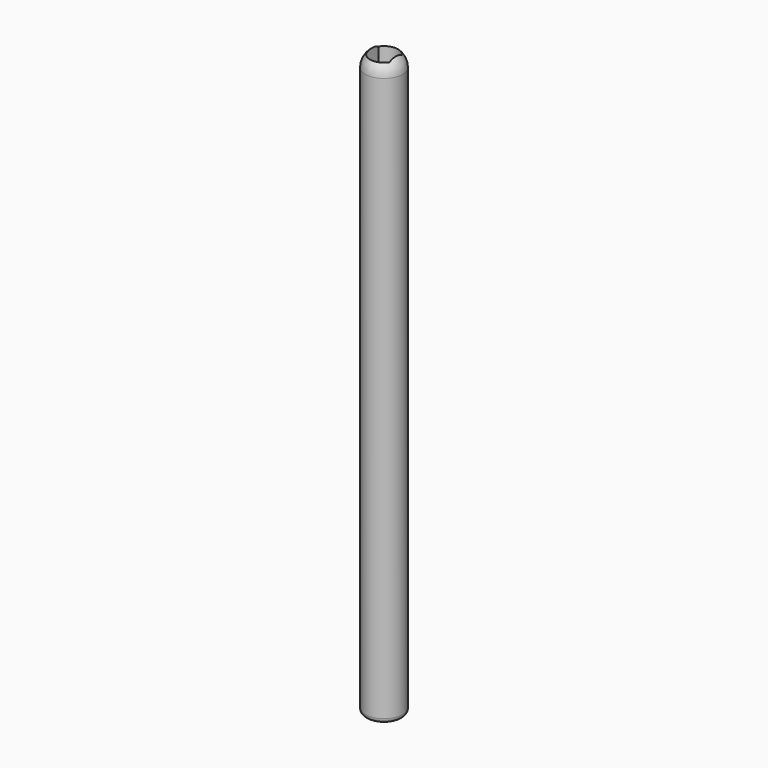
from build123d import *

# Parameters (mm, degrees)
F0_W     = 4
F0_H     = 125
F3_DEPTH = 20
F5_R     = 1


# Not quite as in the source:
# - a fillet or chamfer that OpenCascade refuses, or shapes differently, is made with other operations: its cross-section is extruded or revolved along the edge and cut away or added


with BuildPart() as f1:
    # F0 (on Right) → F1 (revolve)
    with BuildSketch(Plane.YZ):
        with Locations((-2, 0)):
            Rectangle(F0_W, F0_H)
    revolve(axis=Axis((0, 0, 0), (0, 0, -1)))

    # F2 (on face) → F3 (cut)
    with BuildSketch(Plane.XY.offset(62.5)):
        with BuildLine():
            Line((-2.5, 1.6583123952), (-2.5, -1.6583123952))
            ThreePointArc((-2.5, -1.6583123952), (0, -3), (2.5, -1.6583123952))
            Line((2.5, -1.6583123952), (2.5, 1.6583123952))
            ThreePointArc((2.5, 1.6583123952), (0, 3), (-2.5, 1.6583123952))
        make_face()
    extrude(amount=-F3_DEPTH, mode=Mode.SUBTRACT)

    # F4: fillet of radius 3.5 on 1 edges, made by hand

    # F4_s1 → F4_t2 (revolve, cut)
    with BuildSketch(Plane.YZ):
        with BuildLine():
            ThreePointArc((-0.5, 62.5), (-2.9748737342, 61.4748737342), (-4, 59))
            Line((-4, 59), (-4, 62.5))
            Line((-4, 62.5), (-0.5, 62.5))
        make_face()
    revolve(axis=Axis((0, 0, 62.5), (0, 0, -1)), mode=Mode.SUBTRACT)

    # F5
    f5_edges = [f1.edges().sort_by_distance(p)[0] for p in [
        (0, 4, -62.5),
    ]]
    fillet(f5_edges, radius=F5_R)


solid = f1.part
